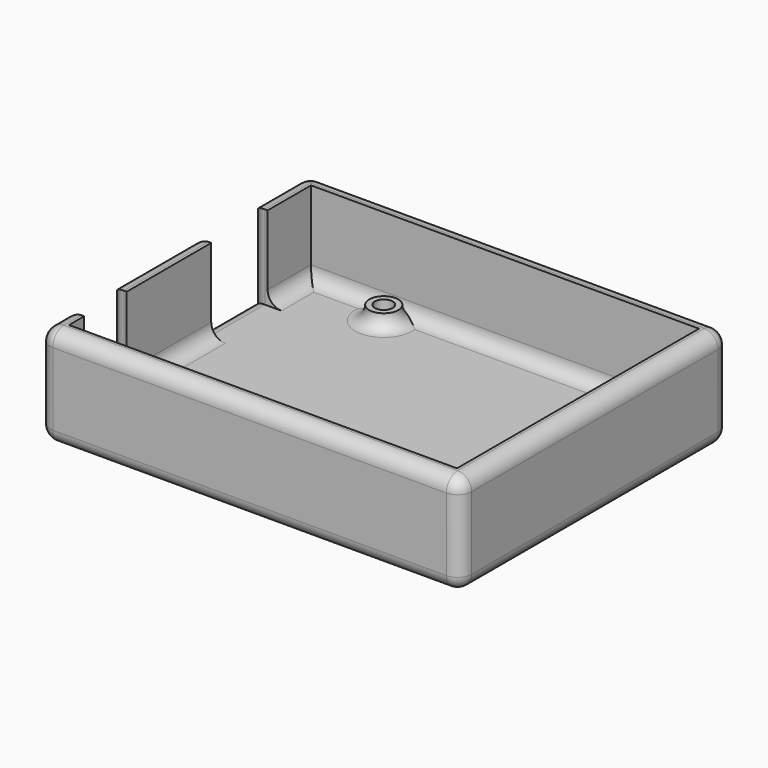
from build123d import *

# Parameters (mm, degrees)
F0_W          = 0.4
F0_H          = 0.3
F0_H_2        = 8.9
F0_W_2        = 9.5
F0_R          = 2.6
F0_W_3        = 10.3
F0_H_3        = 12
F0_W_4        = 3
F0_R_2        = 1.6
F0_H_4        = 18.9
F1_DEPTH      = 3
F2_DEPTH      = 15
F3_DEPTH      = 2.5
F4_T1_DEPTH   = 9.7
F4_T3_DEPTH   = 18.9
F4_T5_DEPTH   = 3.4
F4_T10_DEPTH  = 69.4
F4_S11_R      = 2.6
F4_T12_DEPTH  = 36
F4_T16_DEPTH  = 69.4
F4_S17_R      = 2.6
F4_T18_DEPTH  = 36
F4_T22_DEPTH  = 54.1
F4_S23_R      = 2.6
F4_T24_DEPTH  = 29
F4_S25_R      = 2.6
F4_T26_DEPTH  = 29
F4_T35_DEPTH  = 13
F4_T37_DEPTH  = 21.25
F4_T39_DEPTH  = 12.6
F4_T41_DEPTH  = 9.5
F4_T43_DEPTH  = 55.1
F4_T45_DEPTH  = 70.4
F4_T47_DEPTH  = 31.4
F4_T49_DEPTH  = 16.45
F4_T51_DEPTH  = 10.15
F4_S55_W      = 2.55
F4_S55_H      = 2.55
F4_T56_DEPTH  = 2.55
F4_S61_W      = 2.55
F4_S61_H      = 2.55
F4_T62_DEPTH  = 2.55
F4_S67_W      = 2.55
F4_S67_H      = 2.55
F4_T68_DEPTH  = 2.55
F4_S73_W      = 2.55
F4_S73_H      = 2.55
F4_T74_DEPTH  = 2.55
F4_S79_W      = 2.55
F4_S79_H      = 2.55
F4_T80_DEPTH  = 2.55
F4_S85_W      = 2.55
F4_S85_H      = 2.55
F4_T86_DEPTH  = 2.55
F4_S91_W      = 2.55
F4_S91_H      = 2.55
F4_T92_DEPTH  = 2.55
F4_S97_W      = 2.55
F4_S97_H      = 2.55
F4_T98_DEPTH  = 2.55
F4_T105_DEPTH = 15.75
F4_T109_DEPTH = 21.25
F4_T117_DEPTH = 18.85
F4_T121_DEPTH = 21.25
F4_T129_DEPTH = 21.25
F4_T134_DEPTH = 18.85
F4_T141_DEPTH = 21.25
F4_T146_DEPTH = 15.75
F5_R          = 6.4702703145
F6_DEPTH      = 2.1


# Not quite as in the source:
# - a fillet or chamfer that OpenCascade refuses, or shapes differently, is made with other operations: its cross-section is extruded or revolved along the edge and cut away or added


with BuildPart() as f1:
    # F0 (on Top) → F1 (new body)
    with BuildSketch(Plane.XY):
        Polygon((-34.7, -27.05), (-34.7, -23.65), (-37.7, -23.65), (-37.7, -30.05), (37.7, -30.05), (37.7, 30.05), (-37.7, 30.05), (-37.7, 17.35), (-34.7, 17.35), (-34.7, 27.05), (34.7, 27.05), (34.7, -27.05), align=None)
        with Locations((-34.5, -14.3)):
            Rectangle(F0_W, F0_H)
        with Locations((-34.5, -18.9)):
            Rectangle(F0_W, F0_H_2)
        with Locations((-29.55, -18.9)):
            Rectangle(F0_W_2, F0_H_2)
        Polygon((-34.3, -26.65), (34.3, -26.65), (34.3, 26.65), (-34.3, 26.65), (-34.3, 17.35), (-23.7, 17.35), (-23.7, 4.75), (-34.3, 4.75), (-34.3, -14.15), (-24.5, -14.15), (-24.5, -23.65), (-34.3, -23.65), align=None)
        with Locations((-20.3, -23.85)):
            Circle(F0_R, mode=Mode.SUBTRACT)
        with Locations((31.6, -19.15)):
            Circle(F0_R, mode=Mode.SUBTRACT)
        with Locations((-19.2, 23.95)):
            Circle(F0_R, mode=Mode.SUBTRACT)
        with Locations((31.6, 8.75)):
            Circle(F0_R, mode=Mode.SUBTRACT)
        Polygon((34.3, 26.65), (34.3, -26.65), (-34.3, -26.65), (-34.3, -23.65), (-34.7, -23.65), (-34.7, -27.05), (34.7, -27.05), (34.7, 27.05), (-34.7, 27.05), (-34.7, 17.35), (-34.3, 17.35), (-34.3, 26.65), align=None)
        with Locations((-29.15, 11.05)):
            Rectangle(F0_W_3, F0_H_3)
        with Locations((-36.2, 11.05)):
            Rectangle(F0_W_4, F0_H_3)
        with Locations((-34.5, 11.05)):
            Rectangle(F0_W, F0_H_3)
        with Locations((-36.2, -18.9)):
            Rectangle(F0_W_4, F0_H_2)
        with Locations((-36.2, -14.3)):
            Rectangle(F0_W_4, F0_H)
        with Locations((-19.2, 23.95)):
            Circle(F0_R)
        with Locations((-19.2, 23.95)):
            Circle(F0_R_2, mode=Mode.SUBTRACT)
        with Locations((-20.3, -23.85)):
            Circle(F0_R)
        with Locations((-20.3, -23.85)):
            Circle(F0_R_2, mode=Mode.SUBTRACT)
        with Locations((31.6, -19.15)):
            Circle(F0_R)
        with Locations((31.6, -19.15)):
            Circle(F0_R_2, mode=Mode.SUBTRACT)
        with Locations((31.6, 8.75)):
            Circle(F0_R)
        with Locations((31.6, 8.75)):
            Circle(F0_R_2, mode=Mode.SUBTRACT)
        with Locations((-36.2, 4.9)):
            Rectangle(F0_W_4, F0_H)
        with Locations((-34.5, 4.9)):
            Rectangle(F0_W, F0_H)
        Polygon((-23.7, 17.35), (-34.3, 17.35), (-34.3, 17.05), (-24, 17.05), (-24, 5.05), (-34.3, 5.05), (-34.3, 4.75), (-23.7, 4.75), align=None)
        with Locations((-34.5, -4.7)):
            Rectangle(F0_W, F0_H_4)
        with Locations((-36.2, -4.7)):
            Rectangle(F0_W_4, F0_H_4)
        Polygon((-34.3, -23.35), (-34.3, -23.65), (-24.5, -23.65), (-24.5, -14.15), (-34.3, -14.15), (-34.3, -14.45), (-24.8, -14.45), (-24.8, -23.35), align=None)
        with Locations((-36.2, 17.2)):
            Rectangle(F0_W_4, F0_H)
        with Locations((-34.5, 17.2)):
            Rectangle(F0_W, F0_H)
        with Locations((-34.5, -23.5)):
            Rectangle(F0_W, F0_H)
        with Locations((-36.2, -23.5)):
            Rectangle(F0_W_4, F0_H)
    extrude(amount=-F1_DEPTH)

    # F0 (on Top) → F2 (join)
    with BuildSketch(Plane.XY):
        Polygon((-34.7, -27.05), (-34.7, -23.65), (-37.7, -23.65), (-37.7, -30.05), (37.7, -30.05), (37.7, 30.05), (-37.7, 30.05), (-37.7, 17.35), (-34.7, 17.35), (-34.7, 27.05), (34.7, 27.05), (34.7, -27.05), align=None)
        with Locations((-36.2, -4.7)):
            Rectangle(F0_W_4, F0_H_4)
    extrude(amount=F2_DEPTH)

    # F0 (on Top) → F3 (join)
    with BuildSketch(Plane.XY):
        with Locations((-20.3, -23.85)):
            Circle(F0_R)
        with Locations((-20.3, -23.85)):
            Circle(F0_R_2, mode=Mode.SUBTRACT)
        with Locations((-19.2, 23.95)):
            Circle(F0_R)
        with Locations((-19.2, 23.95)):
            Circle(F0_R_2, mode=Mode.SUBTRACT)
        with Locations((31.6, 8.75)):
            Circle(F0_R)
        with Locations((31.6, 8.75)):
            Circle(F0_R_2, mode=Mode.SUBTRACT)
        with Locations((31.6, -19.15)):
            Circle(F0_R)
        with Locations((31.6, -19.15)):
            Circle(F0_R_2, mode=Mode.SUBTRACT)
    extrude(amount=F3_DEPTH)

    # F4: fillet of radius 2.5 on 30 edges, made by hand

    # F4_s2 → F4_t1 (join)
    with BuildSketch(Plane.XZ.offset(-27.05)):
        with BuildLine():
            ThreePointArc((-34.7, 2.5), (-33.967766953, 0.732233047), (-32.2, 0))
            Line((-32.2, 0), (-34.7, 0))
            Line((-34.7, 0), (-34.7, 2.5))
        make_face()
    extrude(amount=F4_T1_DEPTH)

    # F4_s4 → F4_t3 (join)
    with BuildSketch(Plane.XZ.offset(-4.75)):
        with BuildLine():
            ThreePointArc((-32.2, 0), (-33.967766953, 0.732233047), (-34.7, 2.5))
            Line((-34.7, 2.5), (-34.7, 0))
            Line((-34.7, 0), (-32.2, 0))
        make_face()
    extrude(amount=F4_T3_DEPTH)

    # F4_s6 → F4_t5 (join)
    with BuildSketch(Plane.XZ.offset(23.65)):
        with BuildLine():
            ThreePointArc((-34.7, 2.5), (-33.967766953, 0.732233047), (-32.2, 0))
            Line((-32.2, 0), (-34.7, 0))
            Line((-34.7, 0), (-34.7, 2.5))
        make_face()
    extrude(amount=F4_T5_DEPTH)


with BuildPart() as f4_tool8:
    # F4_s9 → F4_t10 (new body)
    with BuildSketch(Plane.YZ.offset(-34.7)):
        with BuildLine():
            ThreePointArc((27.05, 2.5), (26.317766953, 0.732233047), (24.55, 0))
            Line((24.55, 0), (27.05, 0))
            Line((27.05, 0), (27.05, 2.5))
        make_face()
    extrude(amount=F4_T10_DEPTH)

    # F4_s11 → F4_t12 (cut, symmetric)
    with BuildSketch(Plane.XY.offset(1.2)):
        with Locations((-19.2, 23.95)):
            Circle(F4_S11_R)
    extrude(amount=F4_T12_DEPTH, both=True, mode=Mode.SUBTRACT)


with BuildPart() as f1_1:
    add(f1.part)

    # F4_t7: union F4_tool8
    add(f4_tool8.part)


with BuildPart() as f4_tool14:
    # F4_s15 → F4_t16 (new body)
    with BuildSketch(Plane.YZ.offset(34.7)):
        with BuildLine():
            ThreePointArc((-27.05, 2.5), (-26.317766953, 0.732233047), (-24.55, 0))
            Line((-24.55, 0), (-27.05, 0))
            Line((-27.05, 0), (-27.05, 2.5))
        make_face()
    extrude(amount=-F4_T16_DEPTH)

    # F4_s17 → F4_t18 (cut, symmetric)
    with BuildSketch(Plane.XY.offset(1.2)):
        with Locations((-20.3, -23.85)):
            Circle(F4_S17_R)
    extrude(amount=F4_T18_DEPTH, both=True, mode=Mode.SUBTRACT)


with BuildPart() as f1_2:
    add(f1_1.part)

    # F4_t13: union F4_tool14
    add(f4_tool14.part)


with BuildPart() as f4_tool20:
    # F4_s21 → F4_t22 (new body)
    with BuildSketch(Plane.XZ.offset(-27.05)):
        with BuildLine():
            ThreePointArc((34.7, 2.5), (33.967766953, 0.732233047), (32.2, 0))
            Line((32.2, 0), (34.7, 0))
            Line((34.7, 0), (34.7, 2.5))
        make_face()
    extrude(amount=F4_T22_DEPTH)

    # F4_s23 → F4_t24 (cut, symmetric)
    with BuildSketch(Plane.XY.offset(1.2)):
        with Locations((31.6, -19.15)):
            Circle(F4_S23_R)
    extrude(amount=F4_T24_DEPTH, both=True, mode=Mode.SUBTRACT)

    # F4_s25 → F4_t26 (cut, symmetric)
    with BuildSketch(Plane.XY.offset(1.2)):
        with Locations((31.6, 8.75)):
            Circle(F4_S25_R)
    extrude(amount=F4_T26_DEPTH, both=True, mode=Mode.SUBTRACT)


with BuildPart() as f1_3:
    add(f1_2.part)

    # F4_t19: union F4_tool20
    add(f4_tool20.part)

    # F4_s27 → F4_t28 (revolve)
    with BuildSketch(Plane.XZ.offset(-8.75)):
        with BuildLine():
            ThreePointArc((36.7, 0), (34.932233047, 0.732233047), (34.2, 2.5))
            Line((34.2, 2.5), (34.2, 0))
            Line((34.2, 0), (36.7, 0))
        make_face()
    revolve(axis=Axis((31.6, 8.75, 0), (0, 0, 1)))

    # F4_s29 → F4_t30 (revolve)
    with BuildSketch(Plane.XZ.offset(19.15)):
        with BuildLine():
            ThreePointArc((36.7, 0), (34.932233047, 0.732233047), (34.2, 2.5))
            Line((34.2, 2.5), (34.2, 0))
            Line((34.2, 0), (36.7, 0))
        make_face()
    revolve(axis=Axis((31.6, -19.15, 0), (0, 0, 1)))

    # F4_s31 → F4_t32 (revolve)
    with BuildSketch(Plane.XZ.offset(23.85)):
        with BuildLine():
            ThreePointArc((-15.2, 0), (-16.967766953, 0.732233047), (-17.7, 2.5))
            Line((-17.7, 2.5), (-17.7, 0))
            Line((-17.7, 0), (-15.2, 0))
        make_face()
    revolve(axis=Axis((-20.3, -23.85, 0), (0, 0, 1)))

    # F4_s33 → F4_t34 (revolve)
    with BuildSketch(Plane.XZ.offset(-23.95)):
        with BuildLine():
            ThreePointArc((-14.1, 0), (-15.867766953, 0.732233047), (-16.6, 2.5))
            Line((-16.6, 2.5), (-16.6, 0))
            Line((-16.6, 0), (-14.1, 0))
        make_face()
    revolve(axis=Axis((-19.2, 23.95, 0), (0, 0, 1)))

    # F4_s36 → F4_t35 (cut)
    with BuildSketch(Plane.XY.offset(-0.5)):
        with BuildLine():
            ThreePointArc((35.2, -30.05), (36.967766953, -29.317766953), (37.7, -27.55))
            Line((37.7, -27.55), (37.7, -30.05))
            Line((37.7, -30.05), (35.2, -30.05))
        make_face()
        with BuildLine():
            ThreePointArc((37.7, 27.55), (36.967766953, 29.317766953), (35.2, 30.05))
            Line((35.2, 30.05), (37.7, 30.05))
            Line((37.7, 30.05), (37.7, 27.55))
        make_face()
        with BuildLine():
            ThreePointArc((-37.7, 27.55), (-36.967766953, 29.317766953), (-35.2, 30.05))
            Line((-35.2, 30.05), (-37.7, 30.05))
            Line((-37.7, 30.05), (-37.7, 27.55))
        make_face()
        with BuildLine():
            ThreePointArc((-35.2, -30.05), (-36.967766953, -29.317766953), (-37.7, -27.55))
            Line((-37.7, -27.55), (-37.7, -30.05))
            Line((-37.7, -30.05), (-35.2, -30.05))
        make_face()
    extrude(amount=F4_T35_DEPTH, mode=Mode.SUBTRACT)

    # F4_s38 → F4_t37 (cut)
    with BuildSketch(Plane.XY):
        with BuildLine():
            ThreePointArc((-37.7, -11.65), (-36.967766953, -13.417766953), (-35.2, -14.15))
            Line((-35.2, -14.15), (-37.7, -14.15))
            Line((-37.7, -14.15), (-37.7, -11.65))
        make_face()
        with BuildLine():
            ThreePointArc((-37.7, 19.85), (-36.967766953, 18.082233047), (-35.2, 17.35))
            Line((-35.2, 17.35), (-37.7, 17.35))
            Line((-37.7, 17.35), (-37.7, 19.85))
        make_face()
        with BuildLine():
            ThreePointArc((-37.7, 2.25), (-36.967766953, 4.017766953), (-35.2, 4.75))
            Line((-35.2, 4.75), (-37.7, 4.75))
            Line((-37.7, 4.75), (-37.7, 2.25))
        make_face()
        with BuildLine():
            ThreePointArc((-37.7, -26.15), (-36.967766953, -24.382233047), (-35.2, -23.65))
            Line((-35.2, -23.65), (-37.7, -23.65))
            Line((-37.7, -23.65), (-37.7, -26.15))
        make_face()
    extrude(amount=F4_T37_DEPTH, mode=Mode.SUBTRACT)

    # F4_s40 → F4_t39 (cut)
    with BuildSketch(Plane.XZ.offset(-17.35)):
        with BuildLine():
            ThreePointArc((-37.7, -2.5), (-36.967766953, -0.732233047), (-35.2, 0))
            Line((-35.2, 0), (-37.7, 0))
            Line((-37.7, 0), (-37.7, -2.5))
        make_face()
    extrude(amount=F4_T39_DEPTH, mode=Mode.SUBTRACT)

    # F4_s42 → F4_t41 (cut)
    with BuildSketch(Plane.XZ.offset(14.15)):
        with BuildLine():
            ThreePointArc((-37.7, -2.5), (-36.967766953, -0.732233047), (-35.2, 0))
            Line((-35.2, 0), (-37.7, 0))
            Line((-37.7, 0), (-37.7, -2.5))
        make_face()
    extrude(amount=F4_T41_DEPTH, mode=Mode.SUBTRACT)

    # F4_s44 → F4_t43 (cut)
    with BuildSketch(Plane.XZ.offset(-27.55)):
        with BuildLine():
            ThreePointArc((35.2, -3), (36.967766953, -2.267766953), (37.7, -0.5))
            Line((37.7, -0.5), (37.7, -3))
            Line((37.7, -3), (35.2, -3))
        make_face()
        with BuildLine():
            ThreePointArc((-35.2, -3), (-36.967766953, -2.267766953), (-37.7, -0.5))
            Line((-37.7, -0.5), (-37.7, -3))
            Line((-37.7, -3), (-35.2, -3))
        make_face()
        with BuildLine():
            ThreePointArc((37.7, 12.5), (36.967766953, 14.267766953), (35.2, 15))
            Line((35.2, 15), (37.7, 15))
            Line((37.7, 15), (37.7, 12.5))
        make_face()
    extrude(amount=F4_T43_DEPTH, mode=Mode.SUBTRACT)

    # F4_s46 → F4_t45 (cut)
    with BuildSketch(Plane.YZ.offset(-35.2)):
        with BuildLine():
            ThreePointArc((27.55, -3), (29.317766953, -2.267766953), (30.05, -0.5))
            Line((30.05, -0.5), (30.05, -3))
            Line((30.05, -3), (27.55, -3))
        make_face()
        with BuildLine():
            ThreePointArc((-30.05, -0.5), (-29.317766953, -2.267766953), (-27.55, -3))
            Line((-27.55, -3), (-30.05, -3))
            Line((-30.05, -3), (-30.05, -0.5))
        make_face()
        with BuildLine():
            ThreePointArc((27.55, 15), (29.317766953, 14.267766953), (30.05, 12.5))
            Line((30.05, 12.5), (30.05, 15))
            Line((30.05, 15), (27.55, 15))
        make_face()
        with BuildLine():
            ThreePointArc((-30.05, 12.5), (-29.317766953, 14.267766953), (-27.55, 15))
            Line((-27.55, 15), (-30.05, 15))
            Line((-30.05, 15), (-30.05, 12.5))
        make_face()
    extrude(amount=F4_T45_DEPTH, mode=Mode.SUBTRACT)

    # F4_s48 → F4_t47 (cut)
    with BuildSketch(Plane.XZ.offset(-11)):
        with BuildLine():
            ThreePointArc((-37.7, 12.5), (-36.967766953, 14.267766953), (-35.2, 15))
            Line((-35.2, 15), (-37.7, 15))
            Line((-37.7, 15), (-37.7, 12.5))
        make_face()
    extrude(amount=F4_T47_DEPTH, mode=Mode.SUBTRACT)

    # F4_s50 → F4_t49 (cut)
    with BuildSketch(Plane.XZ.offset(-27.55)):
        with BuildLine():
            ThreePointArc((-35.2, 15), (-36.967766953, 14.267766953), (-37.7, 12.5))
            Line((-37.7, 12.5), (-37.7, 15))
            Line((-37.7, 15), (-35.2, 15))
        make_face()
    extrude(amount=F4_T49_DEPTH, mode=Mode.SUBTRACT)

    # F4_s52 → F4_t51 (cut)
    with BuildSketch(Plane.XZ.offset(17.4)):
        with BuildLine():
            ThreePointArc((-35.2, 15), (-36.967766953, 14.267766953), (-37.7, 12.5))
            Line((-37.7, 12.5), (-37.7, 15))
            Line((-37.7, 15), (-35.2, 15))
        make_face()
    extrude(amount=F4_T51_DEPTH, mode=Mode.SUBTRACT)


with BuildPart() as f4_tool54:
    # F4_s55 → F4_t56 (new body)
    with BuildSketch(Plane.XZ.offset(27.55)):
        with Locations((36.475, -1.775)):
            Rectangle(F4_S55_W, F4_S55_H)
    extrude(amount=F4_T56_DEPTH)

    # F4_s57 → F4_t58 (revolve, cut)
    with BuildSketch(Plane(origin=(35.2, -27.55, -0.5), x_dir=(-0.7071067812, 0, 0.7071067812), z_dir=(0.7071067812, 0, 0.7071067812))):
        with BuildLine():
            ThreePointArc((0, -2.5), (2.5, 0), (0, 2.5))
            Line((0, 2.5), (0, -2.5))
        make_face()
    revolve(axis=Axis((35.2, -27.55, -0.5), (0, -1, 0)), mode=Mode.SUBTRACT)


with BuildPart() as f1_4:
    add(f1_3.part)

    # F4_t53: cut F4_tool54
    add(f4_tool54.part, mode=Mode.SUBTRACT)


with BuildPart() as f4_tool60:
    # F4_s61 → F4_t62 (new body)
    with BuildSketch(Plane.XZ.offset(27.55)):
        with Locations((36.475, 13.775)):
            Rectangle(F4_S61_W, F4_S61_H)
    extrude(amount=F4_T62_DEPTH)

    # F4_s63 → F4_t64 (revolve, cut)
    with BuildSketch(Plane(origin=(35.2, -27.55, 12.5), x_dir=(-0.7071067812, 0, -0.7071067812), z_dir=(-0.7071067812, 0, 0.7071067812))):
        with BuildLine():
            ThreePointArc((0, -2.5), (2.5, 0), (0, 2.5))
            Line((0, 2.5), (0, -2.5))
        make_face()
    revolve(axis=Axis((35.2, -27.55, 12.5), (0, -1, 0)), mode=Mode.SUBTRACT)


with BuildPart() as f1_5:
    add(f1_4.part)

    # F4_t59: cut F4_tool60
    add(f4_tool60.part, mode=Mode.SUBTRACT)


with BuildPart() as f4_tool66:
    # F4_s67 → F4_t68 (new body)
    with BuildSketch(Plane.XY.offset(-0.5)):
        with Locations((36.475, 28.825)):
            Rectangle(F4_S67_W, F4_S67_H)
    extrude(amount=-F4_T68_DEPTH)

    # F4_s69 → F4_t70 (revolve, cut)
    with BuildSketch(Plane(origin=(35.2, 27.55, -0.5), x_dir=(-0.7071067812, -0.7071067812, 0), z_dir=(0.7071067812, -0.7071067812, 0))):
        with BuildLine():
            ThreePointArc((0, -2.5), (2.5, 0), (0, 2.5))
            Line((0, 2.5), (0, -2.5))
        make_face()
    revolve(axis=Axis((35.2, 27.55, -0.5), (0, 0, -1)), mode=Mode.SUBTRACT)


with BuildPart() as f1_6:
    add(f1_5.part)

    # F4_t65: cut F4_tool66
    add(f4_tool66.part, mode=Mode.SUBTRACT)


with BuildPart() as f4_tool72:
    # F4_s73 → F4_t74 (new body)
    with BuildSketch(Plane.YZ.offset(35.2)):
        with Locations((28.825, 13.775)):
            Rectangle(F4_S73_W, F4_S73_H)
    extrude(amount=F4_T74_DEPTH)

    # F4_s75 → F4_t76 (revolve, cut)
    with BuildSketch(Plane(origin=(35.2, 27.55, 12.5), x_dir=(0, -0.7071067812, -0.7071067812), z_dir=(0, -0.7071067812, 0.7071067812))):
        with BuildLine():
            ThreePointArc((0, -2.5), (2.5, 0), (0, 2.5))
            Line((0, 2.5), (0, -2.5))
        make_face()
    revolve(axis=Axis((35.2, 27.55, 12.5), (1, 0, 0)), mode=Mode.SUBTRACT)


with BuildPart() as f1_7:
    add(f1_6.part)

    # F4_t71: cut F4_tool72
    add(f4_tool72.part, mode=Mode.SUBTRACT)


with BuildPart() as f4_tool78:
    # F4_s79 → F4_t80 (new body)
    with BuildSketch(Plane.XY.offset(12.5)):
        with Locations((-36.475, 28.825)):
            Rectangle(F4_S79_W, F4_S79_H)
    extrude(amount=F4_T80_DEPTH)

    # F4_s81 → F4_t82 (revolve, cut)
    with BuildSketch(Plane(origin=(-35.2, 27.55, 12.5), x_dir=(0.7071067812, -0.7071067812, 0), z_dir=(-0.7071067812, -0.7071067812, 0))):
        with BuildLine():
            ThreePointArc((0, -2.5), (2.5, 0), (0, 2.5))
            Line((0, 2.5), (0, -2.5))
        make_face()
    revolve(axis=Axis((-35.2, 27.55, 12.5), (0, 0, 1)), mode=Mode.SUBTRACT)


with BuildPart() as f1_8:
    add(f1_7.part)

    # F4_t77: cut F4_tool78
    add(f4_tool78.part, mode=Mode.SUBTRACT)


with BuildPart() as f4_tool84:
    # F4_s85 → F4_t86 (new body)
    with BuildSketch(Plane.XY.offset(-0.5)):
        with Locations((-36.475, 28.825)):
            Rectangle(F4_S85_W, F4_S85_H)
    extrude(amount=-F4_T86_DEPTH)

    # F4_s87 → F4_t88 (revolve, cut)
    with BuildSketch(Plane(origin=(-35.2, 27.55, -0.5), x_dir=(0.7071067812, -0.7071067812, 0), z_dir=(0.7071067812, 0.7071067812, 0))):
        with BuildLine():
            ThreePointArc((0, -2.5), (2.5, 0), (0, 2.5))
            Line((0, 2.5), (0, -2.5))
        make_face()
    revolve(axis=Axis((-35.2, 27.55, -0.5), (0, 0, -1)), mode=Mode.SUBTRACT)


with BuildPart() as f1_9:
    add(f1_8.part)

    # F4_t83: cut F4_tool84
    add(f4_tool84.part, mode=Mode.SUBTRACT)


with BuildPart() as f4_tool90:
    # F4_s91 → F4_t92 (new body)
    with BuildSketch(Plane.XZ.offset(27.55)):
        with Locations((-36.475, 13.775)):
            Rectangle(F4_S91_W, F4_S91_H)
    extrude(amount=F4_T92_DEPTH)

    # F4_s93 → F4_t94 (revolve, cut)
    with BuildSketch(Plane(origin=(-35.2, -27.55, 12.5), x_dir=(0.7071067812, 0, -0.7071067812), z_dir=(-0.7071067812, 0, -0.7071067812))):
        with BuildLine():
            ThreePointArc((0, -2.5), (2.5, 0), (0, 2.5))
            Line((0, 2.5), (0, -2.5))
        make_face()
    revolve(axis=Axis((-35.2, -27.55, 12.5), (0, -1, 0)), mode=Mode.SUBTRACT)


with BuildPart() as f1_10:
    add(f1_9.part)

    # F4_t89: cut F4_tool90
    add(f4_tool90.part, mode=Mode.SUBTRACT)


with BuildPart() as f4_tool96:
    # F4_s97 → F4_t98 (new body)
    with BuildSketch(Plane.XZ.offset(27.55)):
        with Locations((-36.475, -1.775)):
            Rectangle(F4_S97_W, F4_S97_H)
    extrude(amount=F4_T98_DEPTH)

    # F4_s99 → F4_t100 (revolve, cut)
    with BuildSketch(Plane(origin=(-35.2, -27.55, -0.5), x_dir=(0.7071067812, 0, 0.7071067812), z_dir=(0.7071067812, 0, -0.7071067812))):
        with BuildLine():
            ThreePointArc((0, -2.5), (2.5, 0), (0, 2.5))
            Line((0, 2.5), (0, -2.5))
        make_face()
    revolve(axis=Axis((-35.2, -27.55, -0.5), (0, -1, 0)), mode=Mode.SUBTRACT)


with BuildPart() as f1_11:
    add(f1_10.part)

    # F4_t95: cut F4_tool96
    add(f4_tool96.part, mode=Mode.SUBTRACT)


with BuildPart() as f4_tool103:
    # F4_s104 → F4_t105 (new body)
    with BuildSketch(Plane.XZ.offset(7.9)):
        with BuildLine():
            ThreePointArc((-37.7, -2.5), (-36.967766953, -0.732233047), (-35.2, 0))
            Line((-35.2, 0), (-37.7, 0))
            Line((-37.7, 0), (-37.7, -2.5))
        make_face()
    extrude(amount=F4_T105_DEPTH)

    split(bisect_by=Plane.XZ.offset(14.15), keep=Keep.BOTTOM)


with BuildPart() as f4_tool107:
    # F4_s108 → F4_t109 (new body)
    with BuildSketch(Plane.XY.offset(-6.25)):
        with BuildLine():
            ThreePointArc((-37.7, -11.65), (-36.967766953, -13.417766953), (-35.2, -14.15))
            Line((-35.2, -14.15), (-37.7, -14.15))
            Line((-37.7, -14.15), (-37.7, -11.65))
        make_face()
    extrude(amount=F4_T109_DEPTH)

    split(bisect_by=Plane.XY.offset(-3), keep=Keep.TOP)

    split(bisect_by=Plane.XY, keep=Keep.BOTTOM)


with BuildPart() as f4_tool103_1:
    add(f4_tool103.part)

    # F4_t112: intersect F4_tool107
    add(f4_tool107.part, mode=Mode.INTERSECT)


with BuildPart() as f1_12:
    add(f1_11.part)

    # F4_t101: cut F4_tool103
    add(f4_tool103_1.part, mode=Mode.SUBTRACT)


with BuildPart() as f4_tool115:
    # F4_s116 → F4_t117 (new body)
    with BuildSketch(Plane.XZ.offset(-23.6)):
        with BuildLine():
            ThreePointArc((-37.7, -2.5), (-36.967766953, -0.732233047), (-35.2, 0))
            Line((-35.2, 0), (-37.7, 0))
            Line((-37.7, 0), (-37.7, -2.5))
        make_face()
    extrude(amount=F4_T117_DEPTH)

    split(bisect_by=Plane.XZ.offset(-17.35), keep=Keep.BOTTOM)


with BuildPart() as f4_tool119:
    # F4_s120 → F4_t121 (new body)
    with BuildSketch(Plane.XY.offset(-6.25)):
        with BuildLine():
            ThreePointArc((-37.7, 19.85), (-36.967766953, 18.082233047), (-35.2, 17.35))
            Line((-35.2, 17.35), (-37.7, 17.35))
            Line((-37.7, 17.35), (-37.7, 19.85))
        make_face()
    extrude(amount=F4_T121_DEPTH)

    split(bisect_by=Plane.XY.offset(-3), keep=Keep.TOP)

    split(bisect_by=Plane.XY, keep=Keep.BOTTOM)


with BuildPart() as f4_tool115_1:
    add(f4_tool115.part)

    # F4_t124: intersect F4_tool119
    add(f4_tool119.part, mode=Mode.INTERSECT)


with BuildPart() as f1_13:
    add(f1_12.part)

    # F4_t113: cut F4_tool115
    add(f4_tool115_1.part, mode=Mode.SUBTRACT)


with BuildPart() as f4_tool127:
    # F4_s128 → F4_t129 (new body)
    with BuildSketch(Plane.XY.offset(-6.25)):
        with BuildLine():
            ThreePointArc((-37.7, 2.25), (-36.967766953, 4.017766953), (-35.2, 4.75))
            Line((-35.2, 4.75), (-37.7, 4.75))
            Line((-37.7, 4.75), (-37.7, 2.25))
        make_face()
    extrude(amount=F4_T129_DEPTH)

    split(bisect_by=Plane.XY.offset(-3), keep=Keep.TOP)

    split(bisect_by=Plane.XY, keep=Keep.BOTTOM)


with BuildPart() as f4_tool132:
    # F4_s133 → F4_t134 (new body)
    with BuildSketch(Plane.XZ.offset(-17.35)):
        with BuildLine():
            ThreePointArc((-37.7, -2.5), (-36.967766953, -0.732233047), (-35.2, 0))
            Line((-35.2, 0), (-37.7, 0))
            Line((-37.7, 0), (-37.7, -2.5))
        make_face()
    extrude(amount=F4_T134_DEPTH)

    split(bisect_by=Plane.XZ.offset(-4.75), keep=Keep.TOP)


with BuildPart() as f4_tool127_1:
    add(f4_tool127.part)

    # F4_t136: intersect F4_tool132
    add(f4_tool132.part, mode=Mode.INTERSECT)


with BuildPart() as f1_14:
    add(f1_13.part)

    # F4_t125: cut F4_tool127
    add(f4_tool127_1.part, mode=Mode.SUBTRACT)


with BuildPart() as f4_tool139:
    # F4_s140 → F4_t141 (new body)
    with BuildSketch(Plane.XY.offset(-6.25)):
        with BuildLine():
            ThreePointArc((-37.7, -26.15), (-36.967766953, -24.382233047), (-35.2, -23.65))
            Line((-35.2, -23.65), (-37.7, -23.65))
            Line((-37.7, -23.65), (-37.7, -26.15))
        make_face()
    extrude(amount=F4_T141_DEPTH)

    split(bisect_by=Plane.XY.offset(-3), keep=Keep.TOP)

    split(bisect_by=Plane.XY, keep=Keep.BOTTOM)


with BuildPart() as f4_tool144:
    # F4_s145 → F4_t146 (new body)
    with BuildSketch(Plane.XZ.offset(14.15)):
        with BuildLine():
            ThreePointArc((-37.7, -2.5), (-36.967766953, -0.732233047), (-35.2, 0))
            Line((-35.2, 0), (-37.7, 0))
            Line((-37.7, 0), (-37.7, -2.5))
        make_face()
    extrude(amount=F4_T146_DEPTH)

    split(bisect_by=Plane.XZ.offset(23.65), keep=Keep.TOP)


with BuildPart() as f4_tool139_1:
    add(f4_tool139.part)

    # F4_t148: intersect F4_tool144
    add(f4_tool144.part, mode=Mode.INTERSECT)


with BuildPart() as f1_15:
    add(f1_14.part)

    # F4_t137: cut F4_tool139
    add(f4_tool139_1.part, mode=Mode.SUBTRACT)

    # F5 (on face) → F6 (cut)
    with BuildSketch(Plane(origin=(0, 30.05, 0), x_dir=(-1, 0, 0), z_dir=(0, 1, 0))):
        with Locations((0, 6.0658543371)):
            Circle(F5_R)
    extrude(amount=-F6_DEPTH, mode=Mode.SUBTRACT)


solid = f1_15.part
